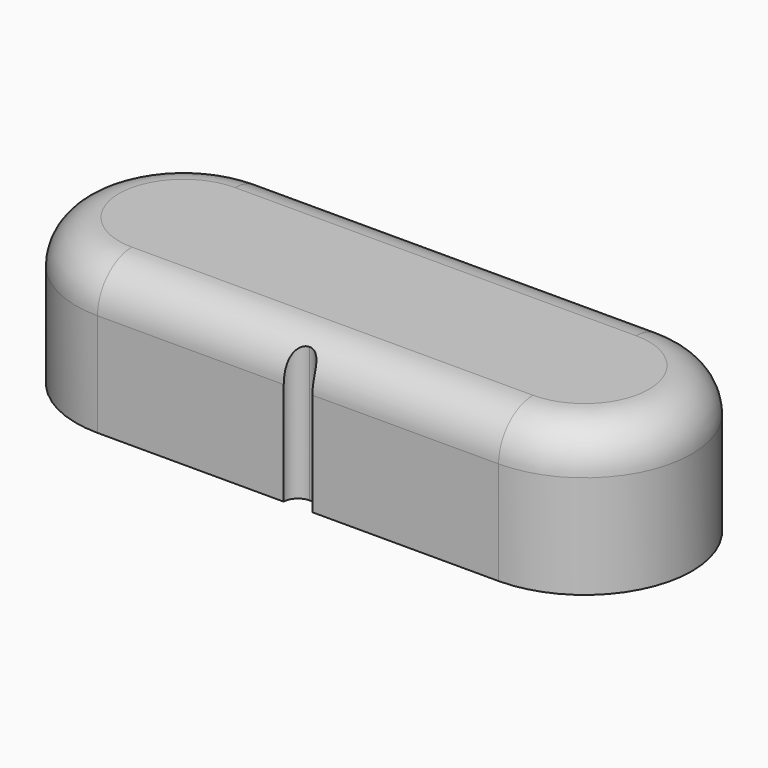
from build123d import *

# Parameters (mm, degrees)
F1_DEPTH    = 51
F2_T1_DEPTH = 102.5
F2_T3_DEPTH = 102.5
F2_T6_ANGLE = 180
F2_T8_ANGLE = 180
F3_T        = -2.5


# Not quite as in the source:
# - a fillet or chamfer that OpenCascade refuses, or shapes differently, is made with other operations: its cross-section is extruded or revolved along the edge and cut away or added


with BuildPart() as f1:
    # F0 (on Top) → F1 (new body)
    with BuildSketch(Plane.XY):
        with BuildLine():
            Line((-70, 37.5), (-70, -37.5))
            Line((-70, -37.5), (-5, -37.5))
            ThreePointArc((-5, -37.5), (-3.5355339059, -33.9644660941), (0, -32.5))
            Line((0, -32.5), (0, 0))
            Line((0, 0), (0, 32.5))
            ThreePointArc((0, 32.5), (-3.5355339059, 33.9644660941), (-5, 37.5))
            Line((-5, 37.5), (-70, 37.5))
        make_face()
        with BuildLine():
            ThreePointArc((-70, 37.5), (-107.5, 0), (-70, -37.5))
            Line((-70, -37.5), (-70, 37.5))
        make_face()
        with BuildLine():
            Line((0, 0), (0, -32.5))
            ThreePointArc((0, -32.5), (3.5355339059, -33.9644660941), (5, -37.5))
            Line((5, -37.5), (70, -37.5))
            Line((70, -37.5), (70, 37.5))
            Line((70, 37.5), (5, 37.5))
            ThreePointArc((5, 37.5), (3.5355339059, 33.9644660941), (0, 32.5))
            Line((0, 32.5), (0, 0))
        make_face()
        with BuildLine():
            Line((70, 37.5), (70, -37.5))
            ThreePointArc((70, -37.5), (107.5, 0), (70, 37.5))
        make_face()
    extrude(amount=F1_DEPTH)

    # F2: fillet of radius 15 on 6 edges, made by hand

    # F2_s2 → F2_t1 (cut)
    with BuildSketch(Plane.YZ.offset(-32.5)):
        with BuildLine():
            ThreePointArc((-37.5, 36), (-33.1066017178, 46.6066017178), (-22.5, 51))
            Line((-22.5, 51), (-37.5, 51))
            Line((-37.5, 51), (-37.5, 36))
        make_face()
        with BuildLine():
            ThreePointArc((37.5, 36), (33.1066017178, 46.6066017178), (22.5, 51))
            Line((22.5, 51), (37.5, 51))
            Line((37.5, 51), (37.5, 36))
        make_face()
    extrude(amount=F2_T1_DEPTH, mode=Mode.SUBTRACT)

    # F2_s4 → F2_t3 (cut)
    with BuildSketch(Plane.YZ.offset(-70)):
        with BuildLine():
            ThreePointArc((37.5, 36), (33.1066017178, 46.6066017178), (22.5, 51))
            Line((22.5, 51), (37.5, 51))
            Line((37.5, 51), (37.5, 36))
        make_face()
        with BuildLine():
            ThreePointArc((-37.5, 36), (-33.1066017178, 46.6066017178), (-22.5, 51))
            Line((-22.5, 51), (-37.5, 51))
            Line((-37.5, 51), (-37.5, 36))
        make_face()
    extrude(amount=F2_T3_DEPTH, mode=Mode.SUBTRACT)

    # F2_s5 → F2_t6 (revolve, cut)
    with BuildSketch(Plane.YZ.offset(70)):
        with BuildLine():
            ThreePointArc((-37.5, 36), (-33.1066017178, 46.6066017178), (-22.5, 51))
            Line((-22.5, 51), (-37.5, 51))
            Line((-37.5, 51), (-37.5, 36))
        make_face()
    revolve(axis=Axis((70, 0, 51), (0, 0, 1)), revolution_arc=F2_T6_ANGLE, mode=Mode.SUBTRACT)

    # F2_s7 → F2_t8 (revolve, cut)
    with BuildSketch(Plane.YZ.offset(-70)):
        with BuildLine():
            ThreePointArc((37.5, 36), (33.1066017178, 46.6066017178), (22.5, 51))
            Line((22.5, 51), (37.5, 51))
            Line((37.5, 51), (37.5, 36))
        make_face()
    revolve(axis=Axis((-70, 0, 51), (0, 0, 1)), revolution_arc=F2_T8_ANGLE, mode=Mode.SUBTRACT)

    # F3
    f3_openings = [f1.faces().sort_by_distance(p)[0] for p in [
        (0, 0, 0),
    ]]
    offset(amount=F3_T, openings=f3_openings)


solid = f1.part
